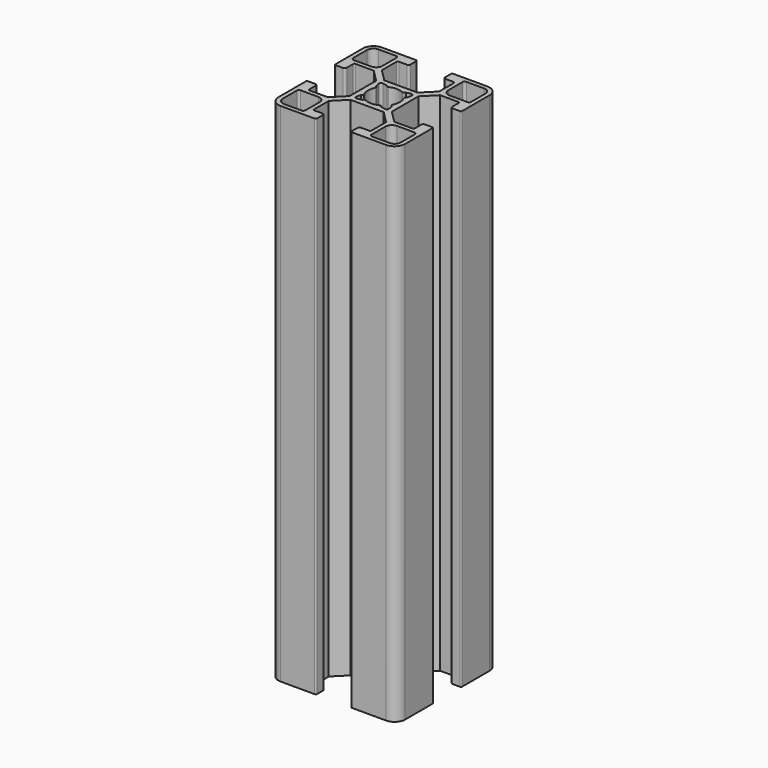
from build123d import *

# Parameters (mm, degrees)
F1_DEPTH = 120


# Not quite as in the source:
# - ends of sketch curves that miss each other by under 0.0002 mm in the source are joined
# - the program builds the solid bodies; features that only make, move or delete a surface that nothing else refers to are left out


with BuildPart() as f1:
    # F0 (on Top) → F1 (new body)
    with BuildSketch(Plane.XY):
        with BuildLine():
            Line((3.939341, -5), (6.799995, -7.860656))
            Line((6.799995, -7.860656), (6.799995, -12.199997))
            ThreePointArc((6.799995, -12.199997), (6.7121307415, -12.4121300846), (6.5, -12.5))
            Line((6.5, -12.5), (4.599998, -12.5))
            ThreePointArc((4.599998, -12.5), (4.2464446094, -12.6464466094), (4.099998, -13))
            Line((4.099998, -13), (4.099998, -14.699997))
            ThreePointArc((4.099998, -14.699997), (4.1878632585, -14.9121300846), (4.399994, -15))
            Line((4.399994, -15), (12.5, -15))
            ThreePointArc((12.5, -15), (14.267766953, -14.267766953), (15, -12.5))
            Line((15, -12.5), (15, -4.399994))
            ThreePointArc((15, -4.399994), (14.9121300846, -4.1878632585), (14.699997, -4.099999))
            Line((14.699997, -4.099999), (13, -4.099998))
            ThreePointArc((13, -4.099998), (12.6464466094, -4.2464446094), (12.5, -4.599998))
            Line((12.5, -4.599998), (12.5, -6.5))
            ThreePointArc((12.5, -6.5), (12.4121300846, -6.7121307415), (12.199997, -6.799995))
            Line((12.199997, -6.799995), (7.860655, -6.799995))
            Line((7.860655, -6.799995), (5, -3.93934))
            Line((5, -3.93934), (5, 3.939341))
            Line((5, 3.939341), (7.860655, 6.799995))
            Line((7.860655, 6.799995), (12.199997, 6.799995))
            ThreePointArc((12.199997, 6.799995), (12.4121300846, 6.7121307415), (12.5, 6.5))
            Line((12.5, 6.5), (12.5, 4.599998))
            ThreePointArc((12.5, 4.599998), (12.6464466094, 4.2464446094), (13, 4.099998))
            Line((13, 4.099998), (14.699997, 4.099998))
            ThreePointArc((14.699997, 4.099998), (14.9121300846, 4.1878632585), (15, 4.399994))
            Line((15, 4.399994), (15, 12.5))
            ThreePointArc((15, 12.5), (14.267766953, 14.267766953), (12.5, 15))
            Line((12.5, 15), (4.399994, 15))
            ThreePointArc((4.399994, 15), (4.1878632585, 14.9121300846), (4.099999, 14.699997))
            Line((4.099999, 14.699997), (4.099998, 13))
            ThreePointArc((4.099998, 13), (4.2464446094, 12.6464466094), (4.599998, 12.5))
            Line((4.599998, 12.5), (6.5, 12.5))
            ThreePointArc((6.5, 12.5), (6.7121307415, 12.4121300846), (6.799995, 12.199997))
            Line((6.799995, 12.199997), (6.799995, 7.860655))
            Line((6.799995, 7.860655), (3.939341, 5))
            Line((3.939341, 5), (-3.93934, 5))
            Line((-3.93934, 5), (-6.799995, 7.860655))
            Line((-6.799995, 7.860655), (-6.799995, 12.199997))
            ThreePointArc((-6.799995, 12.199997), (-6.7121307415, 12.4121300846), (-6.5, 12.5))
            Line((-6.5, 12.5), (-4.599998, 12.5))
            ThreePointArc((-4.599998, 12.5), (-4.2464446094, 12.6464466094), (-4.099998, 13))
            Line((-4.099998, 13), (-4.099998, 14.699997))
            ThreePointArc((-4.099998, 14.699997), (-4.1878632585, 14.9121300846), (-4.399994, 15))
            Line((-4.399994, 15), (-12.5, 15))
            ThreePointArc((-12.5, 15), (-14.267766953, 14.267766953), (-15, 12.5))
            Line((-15, 12.5), (-15, 4.399994))
            ThreePointArc((-15, 4.399994), (-14.9121300846, 4.1878632585), (-14.699997, 4.099999))
            Line((-14.699997, 4.099999), (-13, 4.099998))
            ThreePointArc((-13, 4.099998), (-12.6464466094, 4.2464446094), (-12.5, 4.599998))
            Line((-12.5, 4.599998), (-12.5, 6.5))
            ThreePointArc((-12.5, 6.5), (-12.4121300846, 6.7121307415), (-12.199997, 6.799995))
            Line((-12.199997, 6.799995), (-7.860656, 6.799995))
            Line((-7.860656, 6.799995), (-5, 3.939341))
            Line((-5, 3.939341), (-5, -3.93934))
            Line((-5, -3.93934), (-7.860656, -6.799995))
            Line((-7.860656, -6.799995), (-12.199997, -6.799995))
            ThreePointArc((-12.199997, -6.799995), (-12.4121300846, -6.7121307415), (-12.5, -6.5))
            Line((-12.5, -6.5), (-12.5, -4.599998))
            ThreePointArc((-12.5, -4.599998), (-12.6464466094, -4.2464446094), (-13, -4.099998))
            Line((-13, -4.099998), (-14.699997, -4.099998))
            ThreePointArc((-14.699997, -4.099998), (-14.9121300846, -4.1878632585), (-15, -4.399994))
            Line((-15, -4.399994), (-15, -12.5))
            ThreePointArc((-15, -12.5), (-14.267766953, -14.267766953), (-12.5, -15))
            Line((-12.5, -15), (-4.399994, -15))
            ThreePointArc((-4.399994, -15), (-4.1878632585, -14.9121300846), (-4.099999, -14.699997))
            Line((-4.099999, -14.699997), (-4.099998, -13))
            ThreePointArc((-4.099998, -13), (-4.2464446094, -12.6464466094), (-4.599998, -12.5))
            Line((-4.599998, -12.5), (-6.5, -12.5))
            ThreePointArc((-6.5, -12.5), (-6.7121307415, -12.4121300846), (-6.799995, -12.199997))
            Line((-6.799995, -12.199997), (-6.799995, -7.860656))
            Line((-6.799995, -7.860656), (-3.93934, -5))
            Line((-3.93934, -5), (3.939341, -5))
        make_face()
        with BuildLine():
            Line((-8.299995, -14), (-12.5, -14))
            ThreePointArc((-12.5, -14), (-13.5606601718, -13.5606601718), (-14, -12.5))
            Line((-14, -12.5), (-14, -8.299995))
            ThreePointArc((-14, -8.299995), (-13.8535533906, -7.9464416094), (-13.5, -7.799995))
            Line((-13.5, -7.799995), (-9.299995, -7.799995))
            ThreePointArc((-9.299995, -7.799995), (-8.2393348282, -8.2393348282), (-7.799995, -9.299995))
            Line((-7.799995, -9.299995), (-7.799995, -13.5))
            ThreePointArc((-7.799995, -13.5), (-7.9464416094, -13.8535533906), (-8.299995, -14))
        make_face(mode=Mode.SUBTRACT)
        with BuildLine():
            Line((12.5, -14), (8.299995, -14))
            ThreePointArc((8.299995, -14), (7.9464416094, -13.8535533906), (7.799995, -13.5))
            Line((7.799995, -13.5), (7.799995, -9.299995))
            ThreePointArc((7.799995, -9.299995), (8.2393348282, -8.2393348282), (9.299995, -7.799995))
            Line((9.299995, -7.799995), (13.5, -7.799995))
            ThreePointArc((13.5, -7.799995), (13.8535533906, -7.9464416094), (14, -8.299995))
            Line((14, -8.299995), (14, -12.5))
            ThreePointArc((14, -12.5), (13.5606601718, -13.5606601718), (12.5, -14))
        make_face(mode=Mode.SUBTRACT)
        with BuildLine():
            Line((3.657288, -2.243073), (3.878887, -3.285876))
            ThreePointArc((3.878887, -3.285876), (3.7433613906, -3.7433613906), (3.2858769836, -3.8788870773))
            Line((3.2858769836, -3.8788870773), (2.243074, -3.657287))
            Line((2.243074, -3.657287), (2.005135, -3.419348))
            ThreePointArc((2.005135, -3.419348), (1.841799908, -3.3354753308), (1.6601868142, -3.3624816237))
            ThreePointArc((1.6601868142, -3.3624816237), (0, -3.75), (-1.6601870383, -3.3624810777))
            ThreePointArc((-1.6601870383, -3.3624810777), (-1.841799908, -3.3354753308), (-2.0051340344, -3.4193479656))
            Line((-2.0051340344, -3.4193479656), (-2.243073, -3.657287))
            Line((-2.243073, -3.657287), (-3.285876, -3.878887))
            ThreePointArc((-3.285876, -3.878887), (-3.7433613906, -3.7433613906), (-3.8788870773, -3.2858769836))
            Line((-3.8788870773, -3.2858769836), (-3.657287, -2.243073))
            Line((-3.657287, -2.243073), (-3.419348, -2.005134))
            ThreePointArc((-3.419348, -2.005134), (-3.3354753308, -1.841799908), (-3.3624816237, -1.6601868142))
            ThreePointArc((-3.3624816237, -1.6601868142), (-3.75, 0), (-3.3624810777, 1.6601870383))
            ThreePointArc((-3.3624810777, 1.6601870383), (-3.3354753883, 1.8418002569), (-3.4193484656, 2.0051345344))
            Line((-3.4193484656, 2.0051345344), (-3.657287, 2.243074))
            Line((-3.657287, 2.243074), (-3.878887, 3.285877))
            ThreePointArc((-3.878887, 3.285877), (-3.7433613906, 3.7433613906), (-3.2858769836, 3.8788870773))
            Line((-3.2858769836, 3.8788870773), (-2.243073, 3.657288))
            Line((-2.243073, 3.657288), (-2.005134, 3.419348))
            ThreePointArc((-2.005134, 3.419348), (-1.8418001264, 3.3354753668), (-1.6601872112, 3.3624814277))
            ThreePointArc((-1.6601872112, 3.3624814277), (0, 3.75), (1.6601870383, 3.3624810777))
            ThreePointArc((1.6601870383, 3.3624810777), (1.8418002569, 3.3354753883), (2.0051345344, 3.4193484656))
            Line((2.0051345344, 3.4193484656), (2.243074, 3.657288))
            Line((2.243074, 3.657288), (3.285877, 3.878887))
            ThreePointArc((3.285877, 3.878887), (3.7433610448, 3.7433617364), (3.8788872806, 3.2858779404))
            Line((3.8788872806, 3.2858779404), (3.657288, 2.243074))
            Line((3.657288, 2.243074), (3.419348, 2.005135))
            ThreePointArc((3.419348, 2.005135), (3.3354753668, 1.8418001264), (3.3624814277, 1.6601872112))
            ThreePointArc((3.3624814277, 1.6601872112), (3.75, 0), (3.3624810777, -1.6601870383))
            ThreePointArc((3.3624810777, -1.6601870383), (3.3354753308, -1.841799908), (3.4193479656, -2.0051340344))
            Line((3.4193479656, -2.0051340344), (3.657288, -2.243073))
        make_face(mode=Mode.SUBTRACT)
        with BuildLine():
            Line((-9.299995, 7.799995), (-13.5, 7.799995))
            ThreePointArc((-13.5, 7.799995), (-13.8535533906, 7.9464416094), (-14, 8.299995))
            Line((-14, 8.299995), (-14, 12.5))
            ThreePointArc((-14, 12.5), (-13.5606601718, 13.5606601718), (-12.5, 14))
            Line((-12.5, 14), (-8.299995, 14))
            ThreePointArc((-8.299995, 14), (-7.9464416094, 13.8535533906), (-7.799995, 13.5))
            Line((-7.799995, 13.5), (-7.799995, 9.299995))
            ThreePointArc((-7.799995, 9.299995), (-8.2393348282, 8.2393348282), (-9.299995, 7.799995))
        make_face(mode=Mode.SUBTRACT)
        with BuildLine():
            Line((13.5, 7.799995), (9.299995, 7.799995))
            ThreePointArc((9.299995, 7.799995), (8.2393348282, 8.2393348282), (7.799995, 9.299995))
            Line((7.799995, 9.299995), (7.799995, 13.5))
            ThreePointArc((7.799995, 13.5), (7.9464416094, 13.8535533906), (8.299995, 14))
            Line((8.299995, 14), (12.5, 14))
            ThreePointArc((12.5, 14), (13.5606601718, 13.5606601718), (14, 12.5))
            Line((14, 12.5), (14, 8.299995))
            ThreePointArc((14, 8.299995), (13.8535533906, 7.9464416094), (13.5, 7.799995))
        make_face(mode=Mode.SUBTRACT)
    extrude(amount=F1_DEPTH)


solid = f1.part
